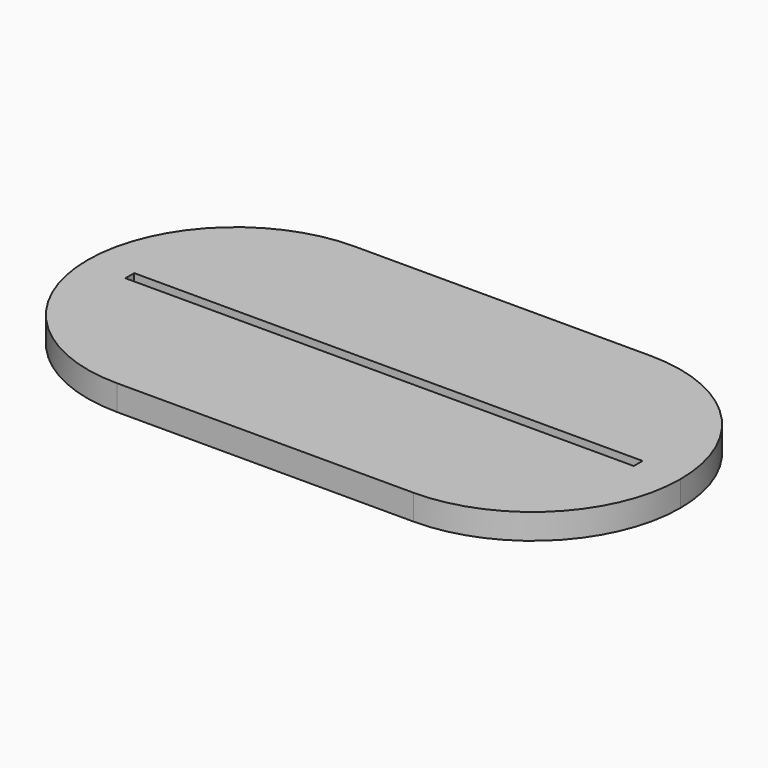
from build123d import *

# Parameters (mm, degrees)
F0_W     = 70
F0_H     = 35
F0_W_2   = 60
F0_H_2   = 1.3
F1_DEPTH = 3
F2_R     = 17.49999
F3_SIZE  = 1


# Not quite as in the source:
# - a fillet or chamfer is up to 0.001 mm smaller than in the source, because OpenCascade refuses the exact size


with BuildPart() as f1:
    # F0 (on Top) → F1 (new body)
    with BuildSketch(Plane.XY):
        with Locations((35, 17.5)):
            Rectangle(F0_W, F0_H)
        with Locations((35, 17.5)):
            Rectangle(F0_W_2, F0_H_2, mode=Mode.SUBTRACT)
    extrude(amount=F1_DEPTH)

    # F2 (radius 17.5 in the source; OpenCascade refuses exactly that, so slightly less here)
    f2_edges = [f1.edges().sort_by_distance(p)[0] for p in [
        (70, 0, 1.5),
        (70, 35, 1.5),
        (0, 35, 1.5),
        (0, 0, 1.5),
    ]]
    fillet(f2_edges, radius=F2_R)

    # F3
    f3_edges = [f1.edges().sort_by_distance(p)[0] for p in [
        (35, 16.85, 0),
        (35, 18.15, 0),
    ]]
    chamfer(f3_edges, length=F3_SIZE)


solid = f1.part
